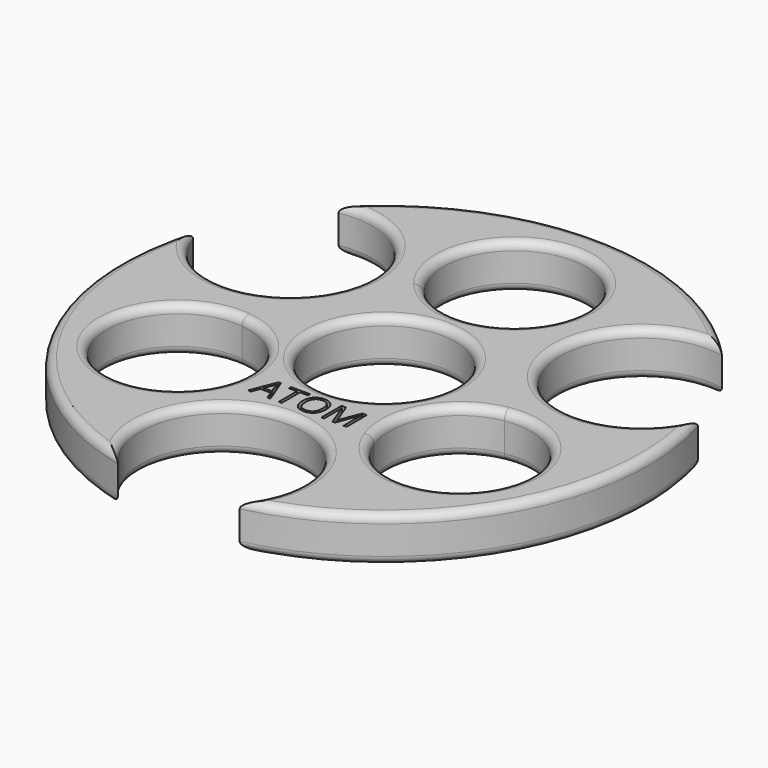
from build123d import *

# Parameters (mm, degrees)
F0_R         = 41.275
F2_DEPTH     = 7
F1_R         = 11.05
F3_DEPTH     = 7
F5_D         = 25.4
F6_R         = 1.27
F7_R         = 1.27
F8_TEXT_SIZE = 5.5555555556
F9_DEPTH     = 1


# Not quite as in the source:
# - Text() gives the source's letters only with a copy of the font that has no kerning and outlines rounded to 1/6400 em; it was checked with that copy


with BuildPart() as f2:
    # F0 (on Top) → F2 (new body)
    with BuildSketch(Plane.XY):
        Circle(F0_R)
        Polygon((-0.0418038421, 33.1022357606), (28.6882790118, -16.514914691), (-28.6464751697, -16.5873210696), align=None, mode=Mode.SUBTRACT)
        Polygon((-28.6464751697, -16.5873210696), (28.6882790118, -16.514914691), (-0.0418038421, 33.1022357606), align=None)
    extrude(amount=F2_DEPTH)

    # F1 (on face) → F3 (cut)
    with BuildSketch(Plane.XY):
        with BuildLine():
            Line((28.6882790118, -16.514914691), (20.1829204723, -1.8260724609))
            ThreePointArc((20.1829204723, -1.8260724609), (12.4341023648, -7.1636550444), (11.607054304, -16.5364860685))
            Line((11.607054304, -16.5364860685), (28.6882790118, -16.514914691))
        make_face()
        with BuildLine():
            ThreePointArc((33.0303299663, -12.7289078311), (29.1301944787, -4.303829941), (20.1829204723, -1.8260724609))
            Line((20.1829204723, -1.8260724609), (28.6882790118, -16.514914691))
            Line((28.6882790118, -16.514914691), (11.607054304, -16.5364860685))
            ThreePointArc((11.607054304, -16.5364860685), (23.913954016, -23.6084114059), (33.0303299663, -12.7289078311))
        make_face()
        Circle(F1_R)
        with BuildLine():
            Line((-28.6464751697, -16.5873210696), (-20.4080066394, -2.2761672884))
            ThreePointArc((-20.4080066394, -2.2761672884), (-30.934032144, -19.2738546033), (-11.1254040764, -16.5651942231))
            Line((-11.1254040764, -16.5651942231), (-28.6464751697, -16.5873210696))
        make_face()
        with BuildLine():
            ThreePointArc((-10.6176703624, -13.2541337351), (-13.4207987089, -5.8994340179), (-20.4080066394, -2.2761672884))
            Line((-20.4080066394, -2.2761672884), (-28.6464751697, -16.5873210696))
            Line((-28.6464751697, -16.5873210696), (-11.1254040764, -16.5651942231))
            ThreePointArc((-11.1254040764, -16.5651942231), (-10.7453413419, -14.9290154533), (-10.6176703624, -13.2541337351))
        make_face()
        with BuildLine():
            Line((-0.0418038421, 33.1022357606), (-8.5237751416, 18.3680900649))
            ThreePointArc((-8.5237751416, 18.3680900649), (-0.0156829676, 14.3500111292), (8.5037804211, 18.3439232892))
            Line((8.5037804211, 18.3439232892), (-0.0418038421, 33.1022357606))
        make_face()
        with BuildLine():
            ThreePointArc((8.5037804211, 18.3439232892), (10.3939711769, 21.6492849784), (11.05, 25.4))
            ThreePointArc((11.05, 25.4), (-3.7359593604, 35.7992839973), (-8.5237751416, 18.3680900649))
            Line((-8.5237751416, 18.3680900649), (-0.0418038421, 33.1022357606))
            Line((-0.0418038421, 33.1022357606), (8.5037804211, 18.3439232892))
        make_face()
    extrude(amount=F3_DEPTH, mode=Mode.SUBTRACT)

    # F5 (through all)
    with Locations(Plane(origin=(0, 0, 0), x_dir=(1, 0, 0), z_dir=(0, 0, -1))):
        with Locations((-27.4343179154, -15.9818866383), (27.5389638759, -15.8008850589), (0, 31.75)):
            Hole(F5_D / 2)

    # F6
    f6_edges = [f2.edges().sort_by_distance(p)[0] for p in [
        (0, -19.05, 7),
        (35.717374, -20.685619, 7),
        (16.523378, 9.480531, 7),
        (0.135899, 41.274776, 7),
        (-16.460591, 9.589132, 7),
        (-35.785288, -20.567906, 7),
        (-32.209937, -9.943073, 7),
        (-11.05, 0, 7),
        (32.353606, -8.92133, 7),
        (-8.50378, 32.456077, 7),
    ]]
    fillet(f6_edges, radius=F6_R)

    # F7
    f7_edges = [f2.edges().sort_by_distance(p)[0] for p in [
        (35.717374, -20.685619, 0),
        (16.523378, 9.480531, 0),
        (0.135899, 41.274776, 0),
        (-16.460591, 9.589132, 0),
        (-35.785288, -20.567906, 0),
        (0, -19.05, 0),
        (-32.209937, -9.943073, 0),
        (-11.05, 0, 0),
        (32.353606, -8.92133, 0),
        (-8.50378, 32.456077, 0),
    ]]
    fillet(f7_edges, radius=F7_R)

    # F8 (on face) → F9 (cut)
    with BuildSketch(Plane.XY.offset(7)):
        with Locations((-7.740327252, -16.9832493271)):
            Text('ATOM', F8_TEXT_SIZE, font='Open Sans', text_align=(TextAlign.LEFT, TextAlign.BOTTOM))
    extrude(amount=-F9_DEPTH, mode=Mode.SUBTRACT)


solid = f2.part
